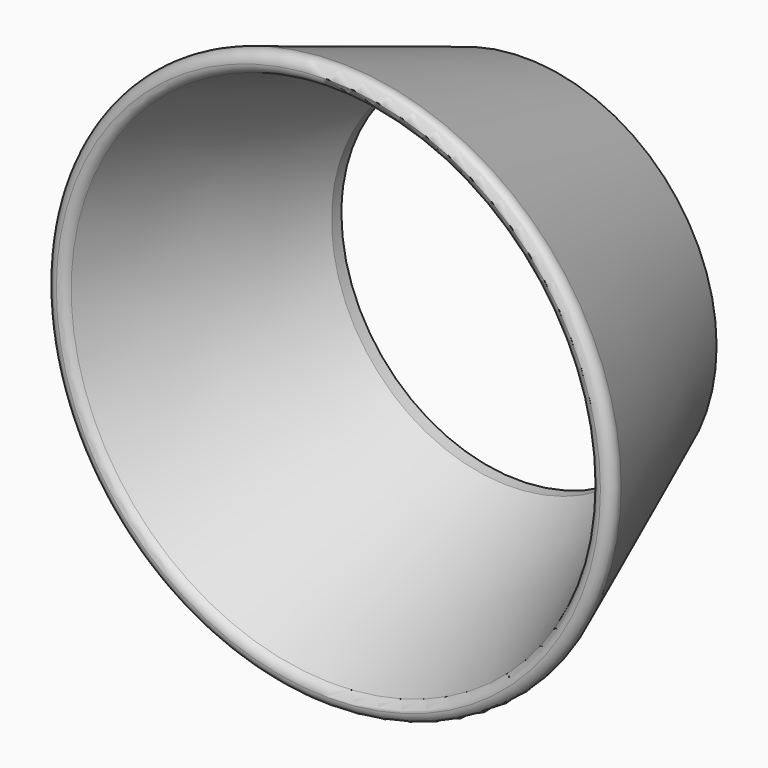
from build123d import *

# Parameters (mm, degrees)
F2_R     = 88.9
F0_R     = 59.26709
F4_T     = -6.35
F5_R     = 54.9232413826
F6_DEPTH = 6.3510001
F7_R     = 3.17499


# Not quite as in the source:
# - a fillet or chamfer is up to 0.001 mm smaller than in the source, because OpenCascade refuses the exact size


with BuildPart() as f3:
    # F2 (on offset) → F3 section 0
    with BuildSketch(Plane.XZ.offset(76.2)):
        Circle(F2_R)
    # F0 (on Front) → F3 section 1
    with BuildSketch(Plane.XZ):
        Circle(F0_R)
    loft()

    # F4
    f4_openings = [f3.faces().sort_by_distance(p)[0] for p in [
        (0, -76.2, 0),
    ]]
    offset(amount=F4_T, openings=f4_openings, kind=Kind.INTERSECTION)

    # F5 (on face) → F6 (cut, through all)
    with BuildSketch(Plane.XZ.offset(6.35)):
        Circle(F5_R)
    extrude(amount=-F6_DEPTH, mode=Mode.SUBTRACT)

    # F7 (radius 3.175 in the source; OpenCascade refuses exactly that, so slightly less here)
    f7_edges = [f3.edges().sort_by_distance(p)[0] for p in [
        (-88.9, -76.2, 0),
        (-82.086742, -76.2, 0),
    ]]
    fillet(f7_edges, radius=F7_R)

    # F8 (on Top) → F9 (revolve, cut)
    with BuildSketch(Plane.XY):
        with BuildLine():
            Line((0, 0), (-59.26709, 0))
            ThreePointArc((-59.26709, 0), (-30.7694079322, -12.346744825), (0, -16.5661673578))
            Line((0, -16.5661673578), (0, 0))
        make_face()
    revolve(axis=Axis((0, -8.2830836789, 0), (0, -1, 0)), mode=Mode.SUBTRACT)


solid = f3.part
